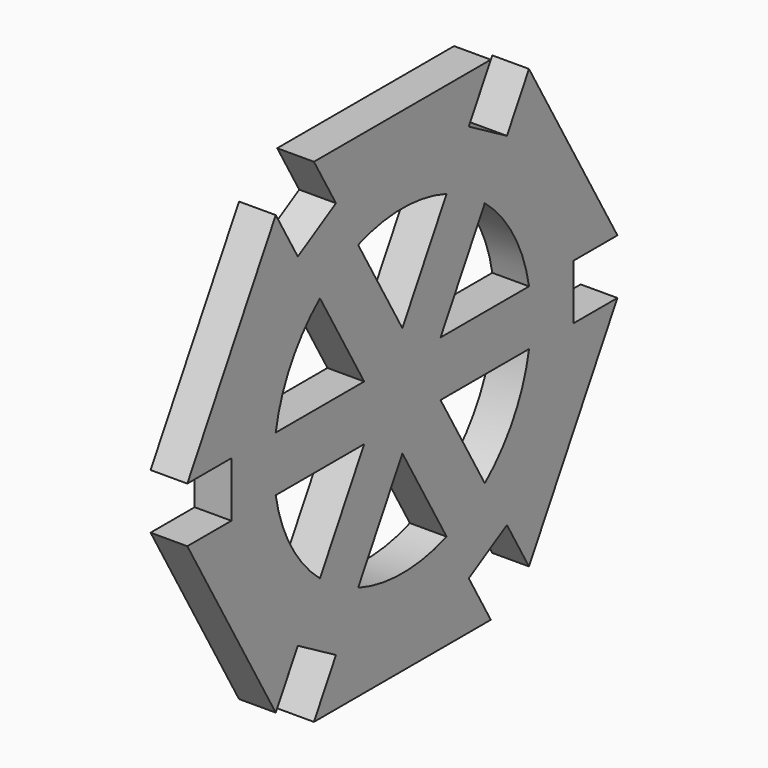
from build123d import *

# Parameters (mm, degrees)
F1_DEPTH = 4


with BuildPart() as f1:
    # F0 (on Right) → F1 (new body)
    with BuildSketch(Plane.YZ):
        Polygon((17.2320508076, -23.8467875173), (29.2679491924, -3), (23.2679491924, -3), (23.2679491924, 3), (29.2679491924, 3), (17.2320508076, 23.8467875173), (14.2320508076, 18.6506350946), (9.0358983849, 21.6506350946), (12.0358983849, 26.8467875173), (-12.0358983849, 26.8467875173), (-9.0358983849, 21.6506350946), (-14.2320508076, 18.6506350946), (-17.2320508076, 23.8467875173), (-29.2679491924, 3), (-23.2679491924, 3), (-23.2679491924, -3), (-29.2679491924, -3), (-17.2320508076, -23.8467875173), (-14.2320508076, -18.6506350946), (-9.0358983849, -21.6506350946), (-12.0358983849, -26.8467875173), (12.0358983849, -26.8467875173), (9.0358983849, -21.6506350946), (14.2320508076, -18.6506350946), align=None)
        with BuildLine():
            ThreePointArc((17.2409396496, 3), (17.4351146235, 1.5055823014), (17.5, 0))
            ThreePointArc((17.5, 0), (17.4351146235, -1.5055823014), (17.2409396496, -3))
            ThreePointArc((17.2409396496, -3), (15.1554445662, -8.75), (11.2185460361, -13.4310917216))
            ThreePointArc((11.2185460361, -13.4310917216), (8.75, -15.1554445662), (6.0223936134, -16.4310917216))
            ThreePointArc((6.0223936134, -16.4310917216), (0, -17.5), (-6.0223936134, -16.4310917216))
            ThreePointArc((-6.0223936134, -16.4310917216), (-8.75, -15.1554445662), (-11.2185460361, -13.4310917216))
            ThreePointArc((-11.2185460361, -13.4310917216), (-15.1554445662, -8.75), (-17.2409396496, -3))
            ThreePointArc((-17.2409396496, -3), (-17.5, 0), (-17.2409396496, 3))
            ThreePointArc((-17.2409396496, 3), (-15.1554445662, 8.75), (-11.2185460361, 13.4310917216))
            ThreePointArc((-11.2185460361, 13.4310917216), (-8.75, 15.1554445662), (-6.0223936134, 16.4310917216))
            ThreePointArc((-6.0223936134, 16.4310917216), (0, 17.5), (6.0223936134, 16.4310917216))
            ThreePointArc((6.0223936134, 16.4310917216), (8.75, 15.1554445662), (11.2185460361, 13.4310917216))
            ThreePointArc((11.2185460361, 13.4310917216), (15.1554445662, 8.75), (17.2409396496, 3))
        make_face(mode=Mode.SUBTRACT)
        with BuildLine():
            ThreePointArc((17.2409396496, -3), (17.4351146235, -1.5055823014), (17.5, 0))
            ThreePointArc((17.5, 0), (17.4351146235, 1.5055823014), (17.2409396496, 3))
            Line((17.2409396496, 3), (5.1961524227, 3))
            Line((5.1961524227, 3), (3.4641016151, 0))
            Line((3.4641016151, 0), (5.1961524227, -3))
            Line((5.1961524227, -3), (17.2409396496, -3))
        make_face()
        with BuildLine():
            Line((5.1961524227, 3), (11.2185460361, 13.4310917216))
            ThreePointArc((11.2185460361, 13.4310917216), (8.75, 15.1554445662), (6.0223936134, 16.4310917216))
            Line((6.0223936134, 16.4310917216), (0, 6))
            Line((0, 6), (1.7320508076, 3))
            Line((1.7320508076, 3), (5.1961524227, 3))
        make_face()
        Polygon((3.4641016151, 0), (5.1961524227, 3), (1.7320508076, 3), align=None)
        with BuildLine():
            ThreePointArc((6.0223936134, -16.4310917216), (8.75, -15.1554445662), (11.2185460361, -13.4310917216))
            Line((11.2185460361, -13.4310917216), (5.1961524227, -3))
            Line((5.1961524227, -3), (1.7320508076, -3))
            Line((1.7320508076, -3), (0, -6))
            Line((0, -6), (6.0223936134, -16.4310917216))
        make_face()
        Polygon((1.7320508076, -3), (5.1961524227, -3), (3.4641016151, 0), align=None)
        Polygon((-1.7320508076, 3), (1.7320508076, 3), (0, 6), align=None)
        Polygon((3.4641016151, 0), (1.7320508076, 3), (-1.7320508076, 3), (-3.4641016151, 0), (-1.7320508076, -3), (1.7320508076, -3), align=None)
        Polygon((0, -6), (1.7320508076, -3), (-1.7320508076, -3), align=None)
        with BuildLine():
            Line((0, 6), (-6.0223936134, 16.4310917216))
            ThreePointArc((-6.0223936134, 16.4310917216), (-8.75, 15.1554445662), (-11.2185460361, 13.4310917216))
            Line((-11.2185460361, 13.4310917216), (-5.1961524227, 3))
            Line((-5.1961524227, 3), (-1.7320508076, 3))
            Line((-1.7320508076, 3), (0, 6))
        make_face()
        Polygon((-3.4641016151, 0), (-1.7320508076, 3), (-5.1961524227, 3), align=None)
        with BuildLine():
            ThreePointArc((-11.2185460361, -13.4310917216), (-8.75, -15.1554445662), (-6.0223936134, -16.4310917216))
            Line((-6.0223936134, -16.4310917216), (0, -6))
            Line((0, -6), (-1.7320508076, -3))
            Line((-1.7320508076, -3), (-5.1961524227, -3))
            Line((-5.1961524227, -3), (-11.2185460361, -13.4310917216))
        make_face()
        Polygon((-5.1961524227, -3), (-1.7320508076, -3), (-3.4641016151, 0), align=None)
        with BuildLine():
            Line((-3.4641016151, 0), (-5.1961524227, 3))
            Line((-5.1961524227, 3), (-17.2409396496, 3))
            ThreePointArc((-17.2409396496, 3), (-17.5, 0), (-17.2409396496, -3))
            Line((-17.2409396496, -3), (-5.1961524227, -3))
            Line((-5.1961524227, -3), (-3.4641016151, 0))
        make_face()
    extrude(amount=F1_DEPTH)


solid = f1.part
